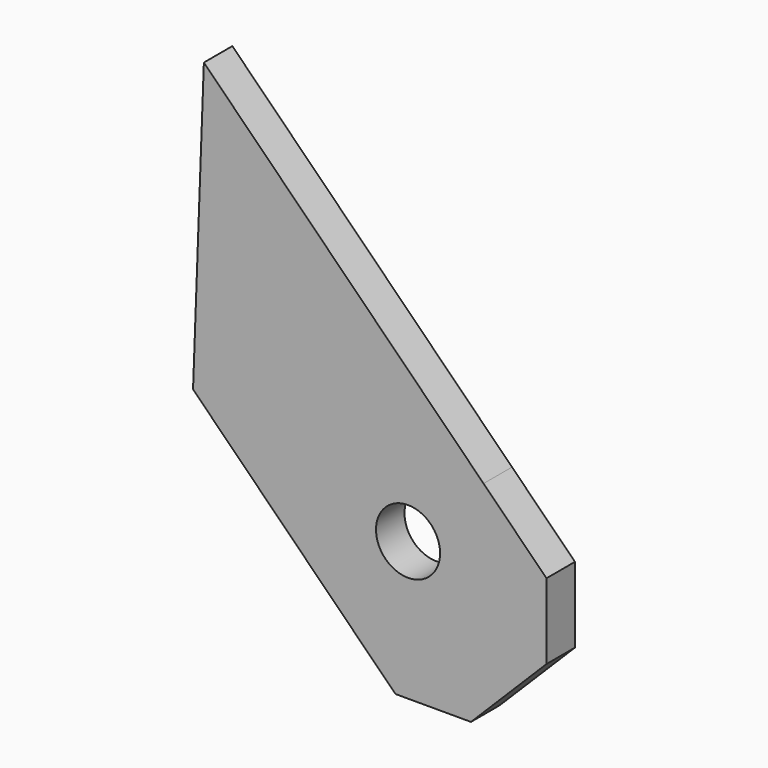
from build123d import *

# Parameters (mm, degrees)
F0_R     = 9
F1_DEPTH = 10
F2_SIZE  = 15


with BuildPart() as f1:
    # F0 (on Front) → F1 (new body)
    with BuildSketch(Plane.XZ):
        Polygon((106.8500287361, -307.0710678119), (78.5657574887, -278.7867965644), (0, -200.2210390757), (-3.0413549592, -282.0324978589), (64.4236218649, -349.4974746831), align=None)
        with Locations((57.3525540531, -300)):
            Circle(F0_R, mode=Mode.SUBTRACT)
    extrude(amount=F1_DEPTH)

    # F2
    f2_edges = [f1.edges().sort_by_distance(p)[0] for p in [
        (106.850029, -5, -307.071068),
        (64.423622, -5, -349.497475),
    ]]
    chamfer(f2_edges, length=F2_SIZE)


solid = f1.part
